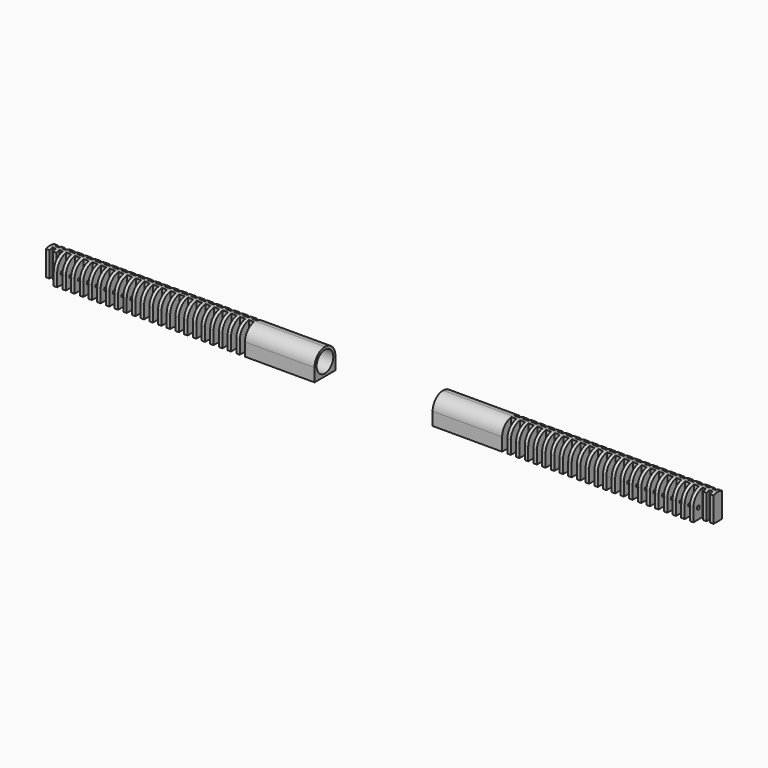
from build123d import *

# Parameters (mm, degrees)
F1_DEPTH  = 15
F2_R      = 7.49999
F3_W      = 3
F3_H      = 10
F4_DEPTH  = 25
F5_R      = 6
F6_DEPTH  = 18
F7_R      = 2.5
F8_DEPTH  = 1.5
F10_R     = 1
F11_DEPTH = 45
F12_R     = 1
F13_DEPTH = 110


# Not quite as in the source:
# - a fillet or chamfer is up to 0.001 mm smaller than in the source, because OpenCascade refuses the exact size


with BuildPart() as f1:
    # F0 (on Top) → F1 (new body)
    with BuildSketch(Plane.XY):
        Polygon((-28.9676572642, -7.5), (-28.9676572642, 7.5), (-178.9676572642, 7.5), (-178.9676572642, 1), (-180.9676572642, 1), (-180.9676572642, 3), (-182.9676572642, 3), (-182.9676572642, 1), (-184.9676572642, 1), (-184.9676572642, 3), (-186.9676572642, 3), (-186.9676572642, 1), (-186.9676572642, -1), (-186.9676572642, -3), (-184.9676572642, -3), (-184.9676572642, -1), (-182.9676572642, -1), (-182.9676572642, -3), (-180.9676572642, -3), (-180.9676572642, -1), (-178.9676572642, -1), (-178.9676572642, -7.5), align=None)
    extrude(amount=F1_DEPTH)

    # F2 (radius 7.5 in the source; OpenCascade refuses exactly that, so slightly less here)
    f2_edges = [f1.edges().sort_by_distance(p)[0] for p in [
        (-103.967657, 7.5, 15),
        (-103.967657, -7.5, 15),
    ]]
    fillet(f2_edges, radius=F2_R)

    # F3 (on Top) → F4 (cut)
    with BuildSketch(Plane.XY):
        with Locations((-70.4676572642, 6)):
            Rectangle(F3_W, F3_H)
        with Locations((-70.4676572642, -6)):
            Rectangle(F3_W, F3_H)
        with Locations((-75.4676572642, 6)):
            Rectangle(F3_W, F3_H)
        with Locations((-75.4676572642, -6)):
            Rectangle(F3_W, F3_H)
        with Locations((-80.4676572642, 6)):
            Rectangle(F3_W, F3_H)
        with Locations((-80.4676572642, -6)):
            Rectangle(F3_W, F3_H)
        with Locations((-85.4676572642, 6)):
            Rectangle(F3_W, F3_H)
        with Locations((-85.4676572642, -6)):
            Rectangle(F3_W, F3_H)
        with Locations((-90.4676572642, 6)):
            Rectangle(F3_W, F3_H)
        with Locations((-90.4676572642, -6)):
            Rectangle(F3_W, F3_H)
        with Locations((-95.4676572642, 6)):
            Rectangle(F3_W, F3_H)
        with Locations((-95.4676572642, -6)):
            Rectangle(F3_W, F3_H)
        with Locations((-100.4676572642, 6)):
            Rectangle(F3_W, F3_H)
        with Locations((-100.4676572642, -6)):
            Rectangle(F3_W, F3_H)
        with Locations((-105.4676572642, 6)):
            Rectangle(F3_W, F3_H)
        with Locations((-105.4676572642, -6)):
            Rectangle(F3_W, F3_H)
        with Locations((-110.4676572642, 6)):
            Rectangle(F3_W, F3_H)
        with Locations((-110.4676572642, -6)):
            Rectangle(F3_W, F3_H)
        with Locations((-115.4676572642, 6)):
            Rectangle(F3_W, F3_H)
        with Locations((-115.4676572642, -6)):
            Rectangle(F3_W, F3_H)
        with Locations((-120.4676572642, 6)):
            Rectangle(F3_W, F3_H)
        with Locations((-120.4676572642, -6)):
            Rectangle(F3_W, F3_H)
        with Locations((-125.4676572642, 6)):
            Rectangle(F3_W, F3_H)
        with Locations((-125.4676572642, -6)):
            Rectangle(F3_W, F3_H)
        with Locations((-130.4676572642, 6)):
            Rectangle(F3_W, F3_H)
        with Locations((-130.4676572642, -6)):
            Rectangle(F3_W, F3_H)
        with Locations((-135.4676572642, 6)):
            Rectangle(F3_W, F3_H)
        with Locations((-135.4676572642, -6)):
            Rectangle(F3_W, F3_H)
        with Locations((-140.4676572642, 6)):
            Rectangle(F3_W, F3_H)
        with Locations((-140.4676572642, -6)):
            Rectangle(F3_W, F3_H)
        with Locations((-145.4676572642, 6)):
            Rectangle(F3_W, F3_H)
        with Locations((-145.4676572642, -6)):
            Rectangle(F3_W, F3_H)
        with Locations((-150.4676572642, 6)):
            Rectangle(F3_W, F3_H)
        with Locations((-150.4676572642, -6)):
            Rectangle(F3_W, F3_H)
        with Locations((-155.4676572642, 6)):
            Rectangle(F3_W, F3_H)
        with Locations((-155.4676572642, -6)):
            Rectangle(F3_W, F3_H)
        with Locations((-160.4676572642, 6)):
            Rectangle(F3_W, F3_H)
        with Locations((-160.4676572642, -6)):
            Rectangle(F3_W, F3_H)
        with Locations((-165.4676572642, 6)):
            Rectangle(F3_W, F3_H)
        with Locations((-165.4676572642, -6)):
            Rectangle(F3_W, F3_H)
        with Locations((-170.4676572642, 6)):
            Rectangle(F3_W, F3_H)
        with Locations((-170.4676572642, -6)):
            Rectangle(F3_W, F3_H)
        with Locations((-175.4676572642, 6)):
            Rectangle(F3_W, F3_H)
        with Locations((-175.4676572642, -6)):
            Rectangle(F3_W, F3_H)
    extrude(amount=F4_DEPTH, mode=Mode.SUBTRACT)

    # F5 (on face) → F6 (cut)
    with BuildSketch(Plane.YZ.offset(-28.9676572642)):
        with Locations((0, 7.5)):
            Circle(F5_R)
    extrude(amount=-F6_DEPTH, mode=Mode.SUBTRACT)

    # F7 (on face) → F8 (cut)
    with BuildSketch(Plane(origin=(0, 7.5, 0), x_dir=(-1, 0, 0), z_dir=(0, 1, 0))):
        with Locations((33.9676572642, 3.75)):
            Circle(F7_R)
        with Locations((63.9676572642, 3.75)):
            Circle(F7_R)
        with Locations((48.9676572642, 3.75)):
            Circle(F7_R)
    extrude(amount=-F8_DEPTH, mode=Mode.SUBTRACT)

    # F10 (on face) → F11 (cut)
    with BuildSketch(Plane(origin=(-178.9676572642, 0, 0), x_dir=(0, -1, 0), z_dir=(-1, 0, 0))):
        with Locations((4, 6)):
            Circle(F10_R)
    extrude(amount=-F11_DEPTH, mode=Mode.SUBTRACT)

    # F12 (on face) → F13 (cut)
    with BuildSketch(Plane(origin=(-178.9676572642, 0, 0), x_dir=(0, -1, 0), z_dir=(-1, 0, 0))):
        with Locations((-4, 6)):
            Circle(F12_R)
    extrude(amount=-F13_DEPTH, mode=Mode.SUBTRACT)


with BuildPart() as f14_1:
    # F14: instance of F1
    add(f1.part.mirror(Plane.YZ.offset(5)))


solid = Compound([f1.part, f14_1.part])
